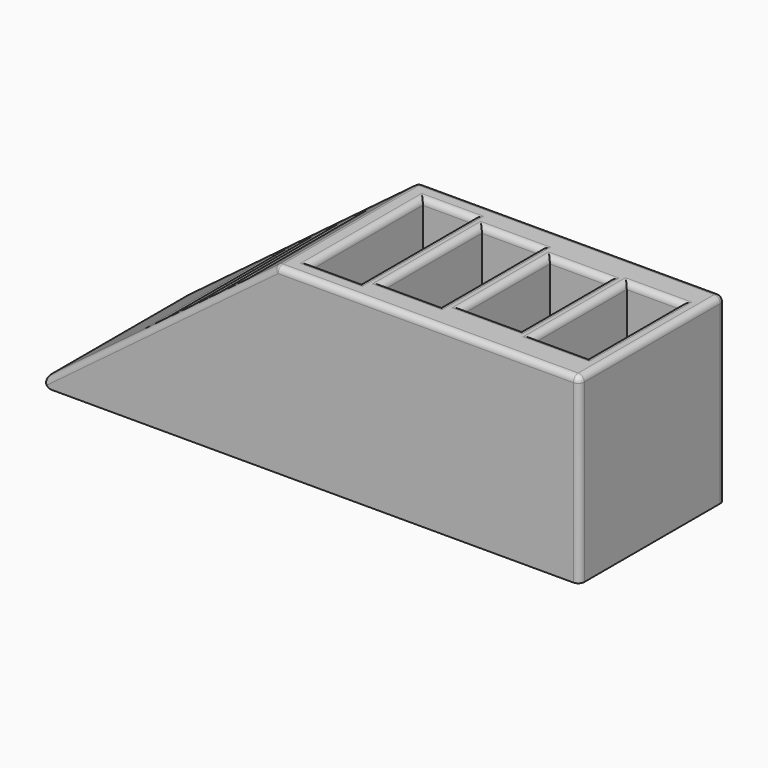
from build123d import *

# Parameters (mm, degrees)
F1_DEPTH = 15
F3_W     = 8.2
F3_H     = 23
F3_W_2   = 9.5
F3_H_2   = 20.3
F3_W_3   = 9.6
F3_H_3   = 17.9
F3_W_4   = 8.9
F3_H_4   = 19.1
F4_DEPTH = 25
F5_W     = 2.5
F5_H     = 24.5
F6_DEPTH = 15
F7_DEPTH = 15
F8_R     = 1


# Not quite as in the source:
# - a feature names something its author has since deleted; it is built from what else it names


with BuildPart() as f1:
    # F0 (on Front) → F1 (new body, symmetric)
    with BuildSketch(Plane.XZ):
        Polygon((25, -15), (25, 15), (-25, 15), (-65, -15), (-25, -15), align=None)
    extrude(amount=F1_DEPTH, both=True)

    # F3 (on offset) → F4 (cut)
    with BuildSketch(Plane.XY.offset(20)):
        with Locations((-17.9062577261, 0)):
            Rectangle(F3_W, F3_H)
        with Locations((-6.4574469417, 0)):
            Rectangle(F3_W_2, F3_H_2)
        with Locations((5.7595338684, 0)):
            Rectangle(F3_W_3, F3_H_3)
        with Locations((17.6052688631, 0)):
            Rectangle(F3_W_4, F3_H_4)
    extrude(amount=-F4_DEPTH, mode=Mode.SUBTRACT)

    # F5 (on face) → F6 (cut)
    with BuildSketch(Plane(origin=(-16.2, 0, 21.6), x_dir=(0.8, 0, 0.6), z_dir=(-0.6, 0, 0.8))):
        with Locations((-20.6918526966, 0)):
            Rectangle(F5_W, F5_H)
    extrude(amount=-F6_DEPTH, mode=Mode.SUBTRACT)

    # F5 (on face) → F7 (cut)
    with BuildSketch(Plane(origin=(-16.2, 0, 21.6), x_dir=(0.8, 0, 0.6), z_dir=(-0.6, 0, 0.8))):
        with Locations((-26.6418426484, -3.204e-07)):
            Rectangle(F5_W, F5_H)
        with Locations((-32.2418349981, 3.204e-07)):
            Rectangle(F5_W, F5_H)
        with Locations((-37.6418220997, 0)):
            Rectangle(F5_W, F5_H)
    extrude(amount=-F7_DEPTH, mode=Mode.SUBTRACT)

    # F8
    f8_edges = [f1.edges().sort_by_distance(p)[0] for p in [
        (-25, 0, 15),
        (-45, 15, 0),
        (-45, -15, 0),
        (-65, 0, -15),
        (-33.753482, 0, 8.434888),
        (-32.753482, 12.25, 9.184888),
        (-32.753482, -12.25, 9.184888),
        (-31.753482, 0, 9.934888),
        (-41.993468, -12.25, 2.254899),
        (-40.993468, 0, 3.004899),
        (-41.993468, 12.25, 2.254899),
        (-42.993468, 0, 1.504899),
        (-45.313458, 0, -0.235093),
        (-46.313458, 12.25, -0.985093),
        (-47.313458, 0, -1.735093),
        (-46.313458, -12.25, -0.985093),
        (-36.513474, 0, 6.364894),
        (-37.513474, 12.25, 5.614894),
        (-38.513474, 0, 4.864894),
        (-37.513474, -12.25, 5.614894),
        (25, 0, 15),
        (0, 15, 15),
        (0, -15, 15),
        (22.055269, 0, 15),
        (17.605269, 9.55, 15),
        (13.155269, 0, 15),
        (17.605269, -9.55, 15),
        (10.559534, 0, 15),
        (5.759534, 8.95, 15),
        (0.959534, 0, 15),
        (5.759534, -8.95, 15),
        (-11.207447, 0, 15),
        (-6.457447, -10.15, 15),
        (-1.707447, 0, 15),
        (-6.457447, 10.15, 15),
        (-17.906258, -11.5, 15),
        (-13.806258, 0, 15),
        (-17.906258, 11.5, 15),
        (-22.006258, 0, 15),
        (25, -15, 0),
        (25, 15, 0),
    ]]
    fillet(f8_edges, radius=F8_R)


solid = f1.part
